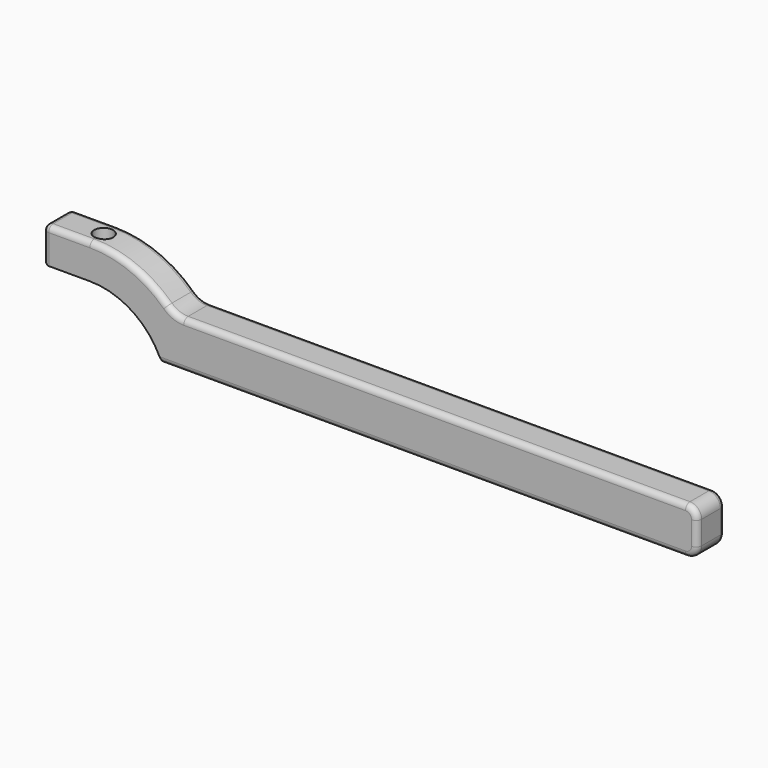
from build123d import *

# Parameters (mm, degrees)
F1_DEPTH     = 4.699
F2_R         = 3.175
F3_R         = 1.524
F4_R         = 6.35
F5_T1_DEPTH  = 11.176
F5_T3_DEPTH  = 136.4146354703
F5_T5_DEPTH  = 6.35
F5_T7_DEPTH  = 146.1327814154
F5_S11_W     = 1.524
F5_S11_H     = 1.524
F5_T12_DEPTH = 1.524
F5_S17_W     = 1.524
F5_S17_H     = 1.524
F5_T18_DEPTH = 1.524
F5_T22_ANGLE = 43.7268911646
F5_T24_ANGLE = 43.7268911646
F5_T26_ANGLE = 90
F5_T28_ANGLE = 90
F5_T30_ANGLE = 43.7268911646
F5_T32_ANGLE = 43.7268911646
F5_T34_ANGLE = 90
F5_T36_ANGLE = 90
F6_R         = 2.5781
F7_DEPTH     = 22.9372001


# Not quite as in the source:
# - a fillet or chamfer that OpenCascade refuses, or shapes differently, is made with other operations: its cross-section is extruded or revolved along the edge and cut away or added


with BuildPart() as f1:
    # F0 (on Front) → F1 (new body, symmetric)
    with BuildSketch(Plane.XZ):
        with BuildLine():
            ThreePointArc((0, 21.0312), (11.8754711368, 17.3575504816), (19.6022185846, 7.62))
            Line((19.6022185846, 7.62), (165.1, 7.62))
            Line((165.1, 7.62), (165.1, 20.32))
            Line((165.1, 20.32), (22.8205819041, 20.32))
            ThreePointArc((22.8205819041, 20.32), (12.5055862406, 27.879951062), (0, 30.5562))
            Line((0, 30.5562), (-12.7, 30.5562))
            Line((-12.7, 30.5562), (-12.7, 21.0312))
            Line((-12.7, 21.0312), (0, 21.0312))
        make_face()
    extrude(amount=F1_DEPTH, both=True)

    # F2
    f2_edges = [f1.edges().sort_by_distance(p)[0] for p in [
        (165.1, 0, 20.32),
        (165.1, 0, 7.62),
    ]]
    fillet(f2_edges, radius=F2_R)

    # F3
    f3_edges = [f1.edges().sort_by_distance(p)[0] for p in [
        (-12.7, 4.699, 25.7937),
        (-12.7, 0, 21.0312),
        (-12.7, -4.699, 25.7937),
        (-12.7, 0, 30.5562),
    ]]
    fillet(f3_edges, radius=F3_R)

    # F4
    f4_edges = [f1.edges().sort_by_distance(p)[0] for p in [
        (22.820582, 0, 20.32),
    ]]
    fillet(f4_edges, radius=F4_R)

    # F5: fillet of radius 1.524 on 2 edges, made by hand

    # F5_s2 → F5_t1 (cut)
    with BuildSketch(Plane.YZ.offset(-11.176)):
        with BuildLine():
            ThreePointArc((-3.175, 30.5562), (-4.2526307345, 30.1098307345), (-4.699, 29.0322))
            Line((-4.699, 29.0322), (-4.699, 30.5562))
            Line((-4.699, 30.5562), (-3.175, 30.5562))
        make_face()
        with BuildLine():
            ThreePointArc((4.699, 29.0322), (4.2526307345, 30.1098307345), (3.175, 30.5562))
            Line((3.175, 30.5562), (4.699, 30.5562))
            Line((4.699, 30.5562), (4.699, 29.0322))
        make_face()
    extrude(amount=F5_T1_DEPTH, mode=Mode.SUBTRACT)

    # F5_s4 → F5_t3 (cut)
    with BuildSketch(Plane.YZ.offset(25.5103645297)):
        with BuildLine():
            ThreePointArc((4.699, 18.796), (4.2526307345, 19.8736307345), (3.175, 20.32))
            Line((3.175, 20.32), (4.699, 20.32))
            Line((4.699, 20.32), (4.699, 18.796))
        make_face()
        with BuildLine():
            ThreePointArc((-3.175, 20.32), (-4.2526307345, 19.8736307345), (-4.699, 18.796))
            Line((-4.699, 18.796), (-4.699, 20.32))
            Line((-4.699, 20.32), (-3.175, 20.32))
        make_face()
    extrude(amount=F5_T3_DEPTH, mode=Mode.SUBTRACT)

    # F5_s6 → F5_t5 (cut)
    with BuildSketch(Plane.XY.offset(10.795)):
        with BuildLine():
            ThreePointArc((163.576, 4.699), (164.6536307345, 4.2526307345), (165.1, 3.175))
            Line((165.1, 3.175), (165.1, 4.699))
            Line((165.1, 4.699), (163.576, 4.699))
        make_face()
        with BuildLine():
            ThreePointArc((165.1, -3.175), (164.6536307345, -4.2526307345), (163.576, -4.699))
            Line((163.576, -4.699), (165.1, -4.699))
            Line((165.1, -4.699), (165.1, -3.175))
        make_face()
    extrude(amount=F5_T5_DEPTH, mode=Mode.SUBTRACT)

    # F5_s8 → F5_t7 (cut)
    with BuildSketch(Plane.YZ.offset(15.7922185846)):
        with BuildLine():
            ThreePointArc((4.699, 9.144), (4.2526307345, 8.0663692655), (3.175, 7.62))
            Line((3.175, 7.62), (4.699, 7.62))
            Line((4.699, 7.62), (4.699, 9.144))
        make_face()
        with BuildLine():
            ThreePointArc((-3.175, 7.62), (-4.2526307345, 8.0663692655), (-4.699, 9.144))
            Line((-4.699, 9.144), (-4.699, 7.62))
            Line((-4.699, 7.62), (-3.175, 7.62))
        make_face()
    extrude(amount=F5_T7_DEPTH, mode=Mode.SUBTRACT)


with BuildPart() as f5_tool10:
    # F5_s11 → F5_t12 (new body)
    with BuildSketch(Plane.XZ.offset(-3.175)):
        with Locations((-11.938, 29.7942)):
            Rectangle(F5_S11_W, F5_S11_H)
    extrude(amount=-F5_T12_DEPTH)

    # F5_s13 → F5_t14 (revolve, cut)
    with BuildSketch(Plane(origin=(-11.176, 3.175, 29.0322), x_dir=(0.7071067812, 0, -0.7071067812), z_dir=(0.7071067812, 0, 0.7071067812))):
        with BuildLine():
            ThreePointArc((0, -1.524), (1.524, 0), (0, 1.524))
            Line((0, 1.524), (0, -1.524))
        make_face()
    revolve(axis=Axis((-11.176, 3.175, 29.0322), (0, 1, 0)), mode=Mode.SUBTRACT)


with BuildPart() as f1_1:
    add(f1.part)

    # F5_t9: cut F5_tool10
    add(f5_tool10.part, mode=Mode.SUBTRACT)


with BuildPart() as f5_tool16:
    # F5_s17 → F5_t18 (new body)
    with BuildSketch(Plane.XY.offset(29.0322)):
        with Locations((-11.938, -3.937)):
            Rectangle(F5_S17_W, F5_S17_H)
    extrude(amount=F5_T18_DEPTH)

    # F5_s19 → F5_t20 (revolve, cut)
    with BuildSketch(Plane(origin=(-11.176, -3.175, 29.0322), x_dir=(0.7071067812, 0.7071067812, 0), z_dir=(0.7071067812, -0.7071067812, 0))):
        with BuildLine():
            ThreePointArc((0, -1.524), (1.524, 0), (0, 1.524))
            Line((0, 1.524), (0, -1.524))
        make_face()
    revolve(axis=Axis((-11.176, -3.175, 29.0322), (0, 0, 1)), mode=Mode.SUBTRACT)


with BuildPart() as f1_2:
    add(f1_1.part)

    # F5_t15: cut F5_tool16
    add(f5_tool16.part, mode=Mode.SUBTRACT)

    # F5_s21 → F5_t22 (revolve, cut)
    with BuildSketch(Plane(origin=(0, 0, 0), x_dir=(0, 1, 0), z_dir=(0.722642808, 0, -0.6912216519))):
        with BuildLine():
            ThreePointArc((4.699, 29.0322), (4.2526307345, 30.1098307345), (3.175, 30.5562))
            Line((3.175, 30.5562), (4.699, 30.5562))
            Line((4.699, 30.5562), (4.699, 29.0322))
        make_face()
    revolve(axis=Axis((0, 4.699, 0), (0, -1, 0)), revolution_arc=F5_T22_ANGLE, mode=Mode.SUBTRACT)

    # F5_s23 → F5_t24 (revolve, cut)
    with BuildSketch(Plane(origin=(0, 0, 0), x_dir=(0, 1, 0), z_dir=(-0.722642808, 0, 0.6912216519))):
        with BuildLine():
            ThreePointArc((4.699, -29.0322), (4.2526307345, -30.1098307345), (3.175, -30.5562))
            Line((3.175, -30.5562), (4.699, -30.5562))
            Line((4.699, -30.5562), (4.699, -29.0322))
        make_face()
    revolve(axis=Axis((25.5103645297, 4.699, 26.67), (0, -1, 0)), revolution_arc=F5_T24_ANGLE, mode=Mode.SUBTRACT)

    # F5_s25 → F5_t26 (revolve, cut)
    with BuildSketch(Plane.YZ.offset(161.925)):
        with BuildLine():
            ThreePointArc((4.699, 18.796), (4.2526307345, 19.8736307345), (3.175, 20.32))
            Line((3.175, 20.32), (4.699, 20.32))
            Line((4.699, 20.32), (4.699, 18.796))
        make_face()
    revolve(axis=Axis((161.925, 4.699, 17.145), (0, 1, 0)), revolution_arc=F5_T26_ANGLE, mode=Mode.SUBTRACT)

    # F5_s27 → F5_t28 (revolve, cut)
    with BuildSketch(Plane.XY.offset(10.795)):
        with BuildLine():
            ThreePointArc((163.576, 4.699), (164.6536307345, 4.2526307345), (165.1, 3.175))
            Line((165.1, 3.175), (165.1, 4.699))
            Line((165.1, 4.699), (163.576, 4.699))
        make_face()
    revolve(axis=Axis((161.925, 4.699, 10.795), (0, 1, 0)), revolution_arc=F5_T28_ANGLE, mode=Mode.SUBTRACT)

    # F5_s29 → F5_t30 (revolve, cut)
    with BuildSketch(Plane(origin=(0, 0, 0), x_dir=(0, 1, 0), z_dir=(0.722642808, 0, -0.6912216519))):
        with BuildLine():
            ThreePointArc((-3.175, 30.5562), (-4.2526307345, 30.1098307345), (-4.699, 29.0322))
            Line((-4.699, 29.0322), (-4.699, 30.5562))
            Line((-4.699, 30.5562), (-3.175, 30.5562))
        make_face()
    revolve(axis=Axis((0, -4.699, 0), (0, -1, 0)), revolution_arc=F5_T30_ANGLE, mode=Mode.SUBTRACT)

    # F5_s31 → F5_t32 (revolve, cut)
    with BuildSketch(Plane(origin=(0, 0, 0), x_dir=(0, 1, 0), z_dir=(-0.722642808, 0, 0.6912216519))):
        with BuildLine():
            ThreePointArc((-3.175, -30.5562), (-4.2526307345, -30.1098307345), (-4.699, -29.0322))
            Line((-4.699, -29.0322), (-4.699, -30.5562))
            Line((-4.699, -30.5562), (-3.175, -30.5562))
        make_face()
    revolve(axis=Axis((25.5103645297, -4.699, 26.67), (0, -1, 0)), revolution_arc=F5_T32_ANGLE, mode=Mode.SUBTRACT)

    # F5_s33 → F5_t34 (revolve, cut)
    with BuildSketch(Plane.YZ.offset(161.925)):
        with BuildLine():
            ThreePointArc((-3.175, 20.32), (-4.2526307345, 19.8736307345), (-4.699, 18.796))
            Line((-4.699, 18.796), (-4.699, 20.32))
            Line((-4.699, 20.32), (-3.175, 20.32))
        make_face()
    revolve(axis=Axis((161.925, -4.699, 17.145), (0, 1, 0)), revolution_arc=F5_T34_ANGLE, mode=Mode.SUBTRACT)

    # F5_s35 → F5_t36 (revolve, cut)
    with BuildSketch(Plane.XY.offset(10.795)):
        with BuildLine():
            ThreePointArc((165.1, -3.175), (164.6536307345, -4.2526307345), (163.576, -4.699))
            Line((163.576, -4.699), (165.1, -4.699))
            Line((165.1, -4.699), (165.1, -3.175))
        make_face()
    revolve(axis=Axis((161.925, -4.699, 10.795), (0, 1, 0)), revolution_arc=F5_T36_ANGLE, mode=Mode.SUBTRACT)

    # F6 (on face) → F7 (cut, through all)
    with BuildSketch(Plane.XY.offset(30.5562)):
        Circle(F6_R)
    extrude(amount=-F7_DEPTH, mode=Mode.SUBTRACT)


solid = f1_2.part
